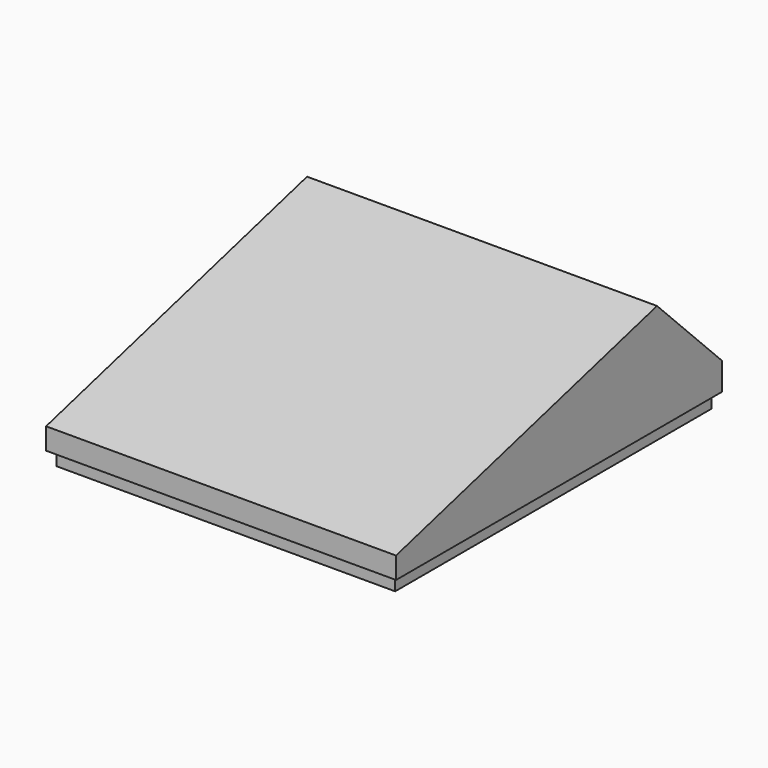
from build123d import *

# Parameters (mm, degrees)
F1_DEPTH      = 77.47
F3_DEPTH      = 1.27
F5_W          = 74.93
F5_H          = 87.551641
F5_W_2        = 72.39
F5_H_2        = 85.011641
F6_DEPTH      = 3.175
F6_DEPTH_BACK = 1.27
F7_W          = 74.93
F7_H          = 24.13
F8_DEPTH      = 9.5758
F10_W         = 74.93
F10_H         = 24.13
F10_W_2       = 70.358
F10_H_2       = 19.558
F11_DEPTH     = 1.905


# Not quite as in the source:
# - a pattern or mirror of a feature is missing from the dataset's text; its kind, count and spacing are read off the source's solid


with BuildPart() as f1:
    # F0 (on Right) → F1 (new body)
    with BuildSketch(Plane.YZ):
        Polygon((88.9000101356, 0), (90.1700101356, 0), (90.1700101356, 6.0914319939), (72.2094978935, 24.0519442361), (0, 4.7625), (0, 0), (1.3483691356, 0), (1.3483691356, 3.8081596938), (71.8294909699, 22.6358999354), (88.9000101356, 5.5653807697), align=None)
    extrude(amount=F1_DEPTH)

    # F2 (on face) → F3 (join)
    with BuildSketch(Plane.YZ.offset(77.47)):
        Polygon((0, 0), (90.1700101356, 0), (90.1700101356, 6.0914319939), (72.2094978935, 24.0519442361), (0, 4.7625), align=None)
    f3 = extrude(amount=-F3_DEPTH)

    # F3_copies: F3 across plane
    add(f3.mirror(Plane(origin=(38.735, 0, 0), x_dir=(0, 0, -1), z_dir=(-1, 0, 0))))

    # F5 (on face) → F6 (join, two sides)
    with BuildSketch(Plane(origin=(0, 0, 0), x_dir=(1, 0, 0), z_dir=(0, 0, -1))) as f6_sk:
        with Locations((38.735, -45.1241896356)):
            Rectangle(F5_W, F5_H)
        with Locations((38.735, -45.1241896356)):
            Rectangle(F5_W_2, F5_H_2, mode=Mode.SUBTRACT)
    extrude(amount=F6_DEPTH)
    extrude(f6_sk.sketch, amount=-F6_DEPTH_BACK)

    # F7 (on face) → F8 (cut)
    with BuildSketch(Plane(origin=(0, 48.1307210648, 48.1307210648), x_dir=(1, 0, 0), z_dir=(0, 0.7071067812, 0.7071067812))):
        with Locations((38.735, 46.7525327565)):
            Rectangle(F7_W, F7_H)
    extrude(amount=-F8_DEPTH, mode=Mode.SUBTRACT)

    # F10 (on offset) → F11 (join)
    with BuildSketch(Plane(origin=(0, 41.3596079495, 41.3596079495), x_dir=(1, 0, 0), z_dir=(0, 0.7071067812, 0.7071067812))):
        with Locations((38.735, 46.7525327565)):
            Rectangle(F10_W, F10_H)
        with Locations((38.735, 46.7525327565)):
            Rectangle(F10_W_2, F10_H_2, mode=Mode.SUBTRACT)
    extrude(amount=-F11_DEPTH)


solid = f1.part
